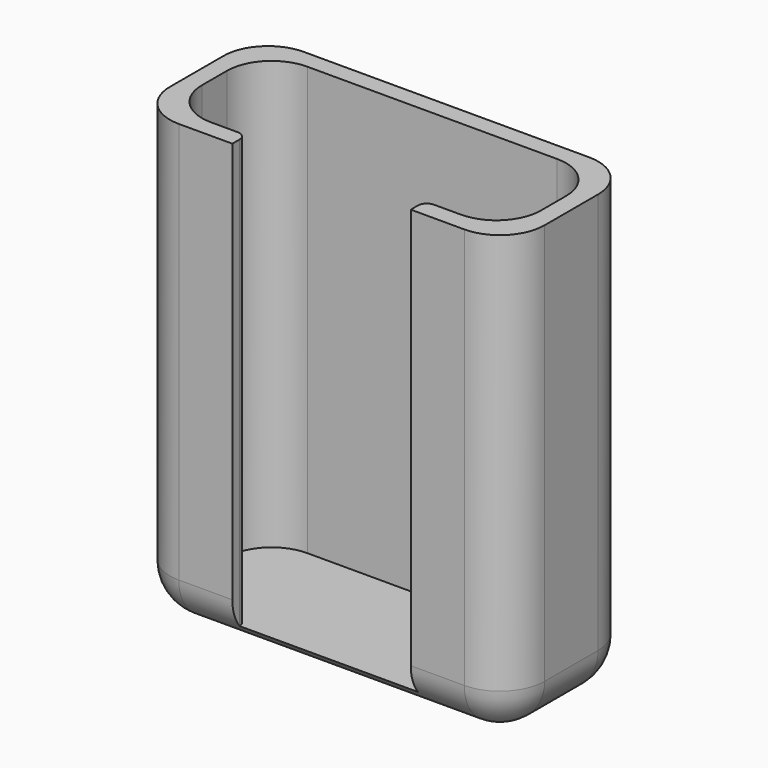
from build123d import *

# Parameters (mm, degrees)
F1_DEPTH     = 50
F0_W         = 20
F0_H         = 2
F2_DEPTH     = 2
F3_T1_DEPTH  = 48
F3_T3_DEPTH  = 57.5
F3_T5_DEPTH  = 32
F3_T7_DEPTH  = 7.5
F3_S11_W     = 5
F3_S11_H     = 5
F3_T12_DEPTH = 5
F3_S17_W     = 5
F3_S17_H     = 5
F3_T18_DEPTH = 5
F3_S23_W     = 5
F3_S23_H     = 5
F3_T24_DEPTH = 5
F3_S29_W     = 5
F3_S29_H     = 5
F3_T30_DEPTH = 5
F4_R         = 1


# Not quite as in the source:
# - a fillet or chamfer that OpenCascade refuses, or shapes differently, is made with other operations: its cross-section is extruded or revolved along the edge and cut away or added


with BuildPart() as f1:
    # F0 (on Top) → F1 (new body)
    with BuildSketch(Plane.XY):
        Polygon((0, 0), (-9, 0), (-9, 13.5), (29, 13.5), (29, 0), (20, 0), (20, -2), (31, -2), (31, 15.5), (-11, 15.5), (-11, -2), (0, -2), align=None)
    extrude(amount=F1_DEPTH)

    # F0 (on Top) → F2 (join)
    with BuildSketch(Plane.XY):
        Polygon((-9, 13.5), (-9, 0), (0, 0), (20, 0), (29, 0), (29, 13.5), align=None)
        with Locations((10, -1)):
            Rectangle(F0_W, F0_H)
    extrude(amount=F2_DEPTH)

    # F3: fillet of radius 5 on 12 edges, made by hand

    # F3_s2 → F3_t1 (join)
    with BuildSketch(Plane.XY.offset(2)):
        with BuildLine():
            ThreePointArc((24, 0), (27.5355339059, 1.4644660941), (29, 5))
            Line((29, 5), (29, 0))
            Line((29, 0), (24, 0))
        make_face()
        with BuildLine():
            ThreePointArc((29, 8.5), (27.5355339059, 12.0355339059), (24, 13.5))
            Line((24, 13.5), (29, 13.5))
            Line((29, 13.5), (29, 8.5))
        make_face()
        with BuildLine():
            ThreePointArc((-4, 0), (-7.5355339059, 1.4644660941), (-9, 5))
            Line((-9, 5), (-9, 0))
            Line((-9, 0), (-4, 0))
        make_face()
        with BuildLine():
            ThreePointArc((-4, 13.5), (-7.5355339059, 12.0355339059), (-9, 8.5))
            Line((-9, 8.5), (-9, 13.5))
            Line((-9, 13.5), (-4, 13.5))
        make_face()
    extrude(amount=F3_T1_DEPTH)

    # F3_s4 → F3_t3 (cut)
    with BuildSketch(Plane.XY.offset(5)):
        with BuildLine():
            ThreePointArc((-6, 15.5), (-9.5355339059, 14.0355339059), (-11, 10.5))
            Line((-11, 10.5), (-11, 15.5))
            Line((-11, 15.5), (-6, 15.5))
        make_face()
        with BuildLine():
            ThreePointArc((-6, -2), (-9.5355339059, -0.5355339059), (-11, 3))
            Line((-11, 3), (-11, -2))
            Line((-11, -2), (-6, -2))
        make_face()
        with BuildLine():
            ThreePointArc((31, 10.5), (29.5355339059, 14.0355339059), (26, 15.5))
            Line((26, 15.5), (31, 15.5))
            Line((31, 15.5), (31, 10.5))
        make_face()
        with BuildLine():
            ThreePointArc((26, -2), (29.5355339059, -0.5355339059), (31, 3))
            Line((31, 3), (31, -2))
            Line((31, -2), (26, -2))
        make_face()
    extrude(amount=F3_T3_DEPTH, mode=Mode.SUBTRACT)

    # F3_s6 → F3_t5 (cut)
    with BuildSketch(Plane.YZ.offset(-6)):
        with BuildLine():
            ThreePointArc((-2, 5), (-0.5355339059, 1.4644660941), (3, 0))
            Line((3, 0), (-2, 0))
            Line((-2, 0), (-2, 5))
        make_face()
        with BuildLine():
            ThreePointArc((15.5, 5), (14.0355339059, 1.4644660941), (10.5, 0))
            Line((10.5, 0), (15.5, 0))
            Line((15.5, 0), (15.5, 5))
        make_face()
    extrude(amount=F3_T5_DEPTH, mode=Mode.SUBTRACT)

    # F3_s8 → F3_t7 (cut)
    with BuildSketch(Plane.XZ.offset(-10.5)):
        with BuildLine():
            ThreePointArc((31, 5), (29.5355339059, 1.4644660941), (26, 0))
            Line((26, 0), (31, 0))
            Line((31, 0), (31, 5))
        make_face()
        with BuildLine():
            ThreePointArc((-11, 5), (-9.5355339059, 1.4644660941), (-6, 0))
            Line((-6, 0), (-11, 0))
            Line((-11, 0), (-11, 5))
        make_face()
    extrude(amount=F3_T7_DEPTH, mode=Mode.SUBTRACT)


with BuildPart() as f3_tool10:
    # F3_s11 → F3_t12 (new body)
    with BuildSketch(Plane.XY.offset(5)):
        with Locations((-8.5, 13)):
            Rectangle(F3_S11_W, F3_S11_H)
    extrude(amount=-F3_T12_DEPTH)

    # F3_s13 → F3_t14 (revolve, cut)
    with BuildSketch(Plane(origin=(-6, 10.5, 5), x_dir=(0.7071067812, -0.7071067812, 0), z_dir=(0.7071067812, 0.7071067812, 0))):
        with BuildLine():
            ThreePointArc((0, -5), (5, 0), (0, 5))
            Line((0, 5), (0, -5))
        make_face()
    revolve(axis=Axis((-6, 10.5, 5), (0, 0, -1)), mode=Mode.SUBTRACT)


with BuildPart() as f1_1:
    add(f1.part)

    # F3_t9: cut F3_tool10
    add(f3_tool10.part, mode=Mode.SUBTRACT)


with BuildPart() as f3_tool16:
    # F3_s17 → F3_t18 (new body)
    with BuildSketch(Plane.XY.offset(5)):
        with Locations((-8.5, 0.5)):
            Rectangle(F3_S17_W, F3_S17_H)
    extrude(amount=-F3_T18_DEPTH)

    # F3_s19 → F3_t20 (revolve, cut)
    with BuildSketch(Plane(origin=(-6, 3, 5), x_dir=(0.7071067812, 0.7071067812, 0), z_dir=(-0.7071067812, 0.7071067812, 0))):
        with BuildLine():
            ThreePointArc((0, -5), (5, 0), (0, 5))
            Line((0, 5), (0, -5))
        make_face()
    revolve(axis=Axis((-6, 3, 5), (0, 0, -1)), mode=Mode.SUBTRACT)


with BuildPart() as f1_2:
    add(f1_1.part)

    # F3_t15: cut F3_tool16
    add(f3_tool16.part, mode=Mode.SUBTRACT)


with BuildPart() as f3_tool22:
    # F3_s23 → F3_t24 (new body)
    with BuildSketch(Plane.XY.offset(5)):
        with Locations((28.5, 13)):
            Rectangle(F3_S23_W, F3_S23_H)
    extrude(amount=-F3_T24_DEPTH)

    # F3_s25 → F3_t26 (revolve, cut)
    with BuildSketch(Plane(origin=(26, 10.5, 5), x_dir=(-0.7071067812, -0.7071067812, 0), z_dir=(0.7071067812, -0.7071067812, 0))):
        with BuildLine():
            ThreePointArc((0, -5), (5, 0), (0, 5))
            Line((0, 5), (0, -5))
        make_face()
    revolve(axis=Axis((26, 10.5, 5), (0, 0, -1)), mode=Mode.SUBTRACT)


with BuildPart() as f1_3:
    add(f1_2.part)

    # F3_t21: cut F3_tool22
    add(f3_tool22.part, mode=Mode.SUBTRACT)


with BuildPart() as f3_tool28:
    # F3_s29 → F3_t30 (new body)
    with BuildSketch(Plane.XY.offset(5)):
        with Locations((28.5, 0.5)):
            Rectangle(F3_S29_W, F3_S29_H)
    extrude(amount=-F3_T30_DEPTH)

    # F3_s31 → F3_t32 (revolve, cut)
    with BuildSketch(Plane(origin=(26, 3, 5), x_dir=(-0.7071067812, 0.7071067812, 0), z_dir=(-0.7071067812, -0.7071067812, 0))):
        with BuildLine():
            ThreePointArc((0, -5), (5, 0), (0, 5))
            Line((0, 5), (0, -5))
        make_face()
    revolve(axis=Axis((26, 3, 5), (0, 0, -1)), mode=Mode.SUBTRACT)


with BuildPart() as f1_4:
    add(f1_3.part)

    # F3_t27: cut F3_tool28
    add(f3_tool28.part, mode=Mode.SUBTRACT)

    # F4
    f4_edges = [f1_4.edges().sort_by_distance(p)[0] for p in [
        (0, 0, 26),
        (20, 0, 26),
    ]]
    fillet(f4_edges, radius=F4_R)


solid = f1_4.part
